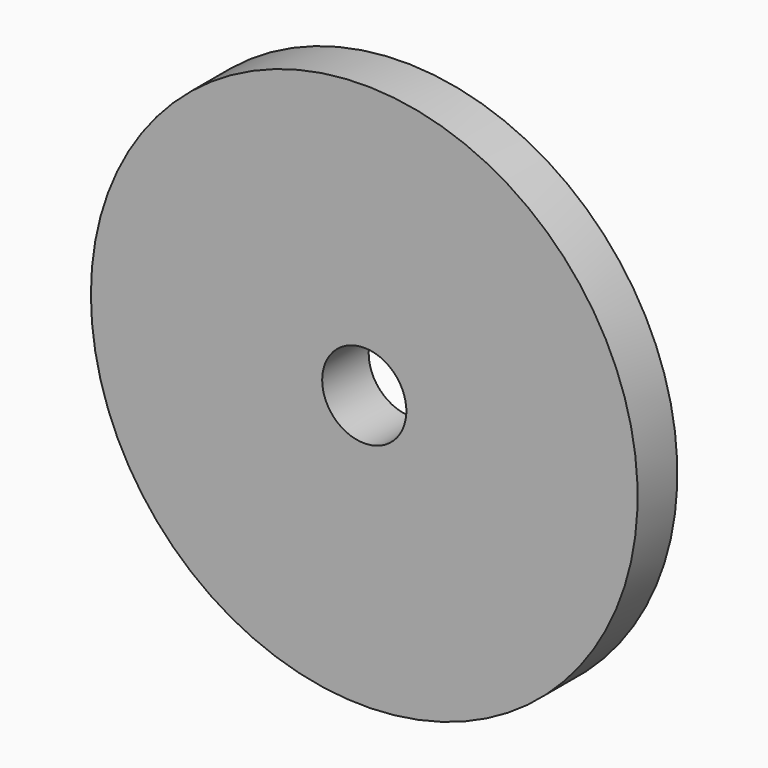
from build123d import *

# Parameters (mm, degrees)
F0_W = 63.45
F0_H = 2.54


# Not quite as in the source:
# - a feature names something its author has since deleted; it is built from what else it names


with BuildPart() as f1:
    # F0 (on Top) → F1 (revolve)
    with BuildSketch(Plane.XY):
        Polygon((-10.8670645285, -41.1176908899), (-17.2170645285, -41.1176908899), (-17.2170645285, -56.1176908899), (52.5829354715, -56.1176908899), (52.5829354715, -41.1176908899), align=None)
        with Locations((20.8579354715, -39.8476908899)):
            Rectangle(F0_W, F0_H)
    revolve(axis=Axis((65.2829354715, -48.6176908899, 0), (0, -1, 0)))


solid = f1.part
